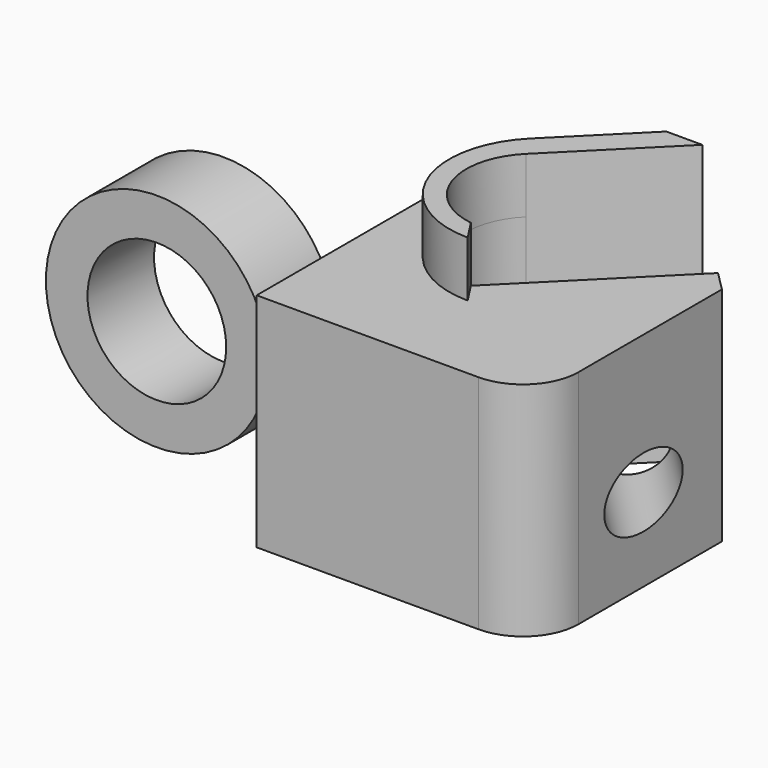
from build123d import *

# Parameters (mm, degrees)
F0_R         = 6.35
F1_DEPTH     = 7.62
F2_W         = 7.62
F2_H         = 6.35
F3_DEPTH     = 25.4
F5_DEPTH     = 25.4
F7_DEPTH     = 63.5
F9_DEPTH     = 20.32
F11_DEPTH    = 25.4
F12_R        = 5.08
F13_R        = 0.508
F14_T1_DEPTH = 46.4482991577
F16_DEPTH    = 5.08
F18_DEPTH    = 1.27
F19_T4_DEPTH = 19.0509661188
F20_R        = 0.254


# Not quite as in the source:
# - a fillet or chamfer that OpenCascade refuses, or shapes differently, is made with other operations: its cross-section is extruded or revolved along the edge and cut away or added


with BuildPart() as f1:
    # F0 (on Front) → F1 (new body)
    with BuildSketch(Plane.XZ):
        with BuildLine():
            Line((15.24, 3.81), (9.4185720786, 3.81))
            ThreePointArc((9.4185720786, 3.81), (-10.16, 0), (9.4185720786, -3.81))
            Line((9.4185720786, -3.81), (15.24, -3.81))
            Line((15.24, -3.81), (15.24, 0))
            Line((15.24, 0), (15.24, 3.81))
        make_face()
        Circle(F0_R, mode=Mode.SUBTRACT)
    extrude(amount=F1_DEPTH)

    # F2 (on face) → F3 (join)
    with BuildSketch(Plane.YZ.offset(15.24)):
        Polygon((-7.62, 10.16), (-7.62, 3.81), (-15.24, 3.81), (-15.24, -10.16), (15.24, -10.16), (15.24, 3.81), (15.24, 10.16), align=None)
        with Locations((-11.43, 6.985)):
            Rectangle(F2_W, F2_H)
    extrude(amount=F3_DEPTH)

    # F4 (on face) → F5 (cut)
    with BuildSketch(Plane.XY.offset(10.16)):
        Polygon((31.65983, 15.24), (40.64, 15.24), (40.64, 6.25983), (47.585287597, 13.2393133827), (38.6222154898, 22.2023854898), align=None)
        Polygon((40.64, 6.25983), (40.64, 15.24), (31.65983, 15.24), align=None)
        with BuildLine():
            Line((40.64, 6.25983), (31.65983, 15.24))
            Line((31.65983, 15.24), (22.6795738789, 6.2597438789))
            ThreePointArc((22.6795738789, 6.2597438789), (22.6795738789, -2.7204261211), (31.6597438789, -2.7204261211))
            Line((31.6597438789, -2.7204261211), (40.64, 6.25983))
        make_face()
    extrude(amount=-F5_DEPTH, mode=Mode.SUBTRACT)

    # F6 (on face) → F7 (cut, symmetric)
    with BuildSketch(Plane(origin=(8.209915, -8.209915, 0), x_dir=(0.7071067812, 0.7071067812, 0), z_dir=(0.7071067812, -0.7071067812, 0))):
        with BuildLine():
            ThreePointArc((26.8131878295, 0.635), (24.5681237992, -4.7850640303), (29.9881878295, -2.54))
            ThreePointArc((29.9881878295, -2.54), (29.0582518598, -0.2949359697), (26.8131878295, 0.635))
        make_face()
    extrude(amount=F7_DEPTH, both=True, mode=Mode.SUBTRACT)

    # F8 (on face) → F9 (join)
    with BuildSketch(Plane.XY.offset(10.16)):
        with BuildLine():
            Line((31.6597438789, -2.7204261211), (40.64, 6.25983))
            Line((40.64, 6.25983), (38.8439487758, 8.0558812242))
            Line((38.8439487758, 8.0558812242), (26.2716117366, -4.516455815))
            ThreePointArc((26.2716117366, -4.516455815), (29.177671493, -4.2544271062), (31.6597438789, -2.7204261211))
        make_face()
    extrude(amount=-F9_DEPTH)

    # F10 (on face) → F11 (cut)
    with BuildSketch(Plane(origin=(8.209915, -8.209915, 0), x_dir=(0.7071067812, 0.7071067812, 0), z_dir=(0.7071067812, -0.7071067812, 0))):
        with BuildLine():
            ThreePointArc((29.9881878295, -2.54), (29.0582518598, -0.2949359697), (26.8131878295, 0.635))
            ThreePointArc((26.8131878295, 0.635), (24.5681237992, -4.7850640303), (29.9881878295, -2.54))
        make_face()
    extrude(amount=F11_DEPTH, mode=Mode.SUBTRACT)

    # F12
    f12_edges = [f1.edges().sort_by_distance(p)[0] for p in [
        (40.64, -15.24, 0),
    ]]
    fillet(f12_edges, radius=F12_R)

    # F13
    f13_edges = [f1.edges().sort_by_distance(p)[0] for p in [
        (15.24, -3.81, 3.81),
        (15.24, -3.81, -3.81),
    ]]
    fillet(f13_edges, radius=F13_R)

    # F14: chamfer of 5.08 on 1 edges, made by hand

    # F14_s2 → F14_t1 (cut)
    with BuildSketch(Plane.XY.offset(-23.2241495789)):
        Polygon((15.24, 10.16), (20.32, 15.24), (15.24, 15.24), align=None)
    extrude(amount=F14_T1_DEPTH, mode=Mode.SUBTRACT)

    # F15 (on face) → F16 (join)
    with BuildSketch(Plane.XY.offset(10.16)):
        with BuildLine():
            Line((31.65983, 15.24), (28.3609535545, 15.24))
            Line((28.3609535545, 15.24), (21.4524150836, 8.3314615291))
            ThreePointArc((21.4524150836, 8.3314615291), (19.5659150525, -1.0873397162), (27.5316145271, -6.4557967708))
            Line((27.5316145271, -6.4557967708), (26.2716117366, -4.516455815))
            ThreePointArc((26.2716117366, -4.516455815), (21.1455728938, -0.2383537351), (22.6795738789, 6.2597438789))
            Line((22.6795738789, 6.2597438789), (31.65983, 15.24))
        make_face()
    extrude(amount=F16_DEPTH)

    # F17 (on face) → F18 (cut)
    with BuildSketch(Plane.XY.offset(10.16)):
        Polygon((21.4524150836, 8.3314615291), (28.3609535545, 15.24), (25.7178656757, 15.24), (19.4216053933, 9.3011604622), align=None)
    extrude(amount=-F18_DEPTH, mode=Mode.SUBTRACT)

    # F19: fillet of radius 5.08 on 1 edges, made by hand


with BuildPart() as f19_tool2:
    # F19_s3 → F19_t4 (new body)
    with BuildSketch(Plane(origin=(4.6185626358, -2.2053347891, 0), x_dir=(0, 0, 1), z_dir=(0.9024034915, -0.4308920265, 0))):
        with BuildLine():
            ThreePointArc((8.89, -20.1221187471), (9.2180951188, -18.3260675229), (10.16, -16.762014582))
            Line((10.16, -16.762014582), (10.0838, -16.6948124987))
            ThreePointArc((10.0838, -16.6948124987), (9.525, -16.660414582), (8.89, -16.660414582))
            Line((8.89, -16.660414582), (8.7884, -16.762014582))
            Line((8.7884, -16.762014582), (8.7884, -20.1221187471))
            Line((8.7884, -20.1221187471), (8.89, -20.1221187471))
        make_face()
    extrude(amount=F19_T4_DEPTH)

    split(bisect_by=Plane(origin=(6.5604767773, -6.5604767773, 0), x_dir=(0, 0, 1), z_dir=(-0.7071067812, 0.7071067812, 0)), keep=Keep.TOP)

    split(bisect_by=Plane(origin=(4.5012786836, -4.7721818404, 0), x_dir=(0, 0, 1), z_dir=(0.6861575418, -0.727452973, 0)), keep=Keep.TOP)


with BuildPart() as f1_1:
    add(f1.part)

    # F19_t1: union F19_tool2
    add(f19_tool2.part)

    # F20
    f20_edges = [f1_1.edges().sort_by_distance(p)[0] for p in [
        (23.880158, 13.506614, 8.89),
        (20.64155, 10.451852, 9.218095),
    ]]
    fillet(f20_edges, radius=F20_R)


solid = f1_1.part
